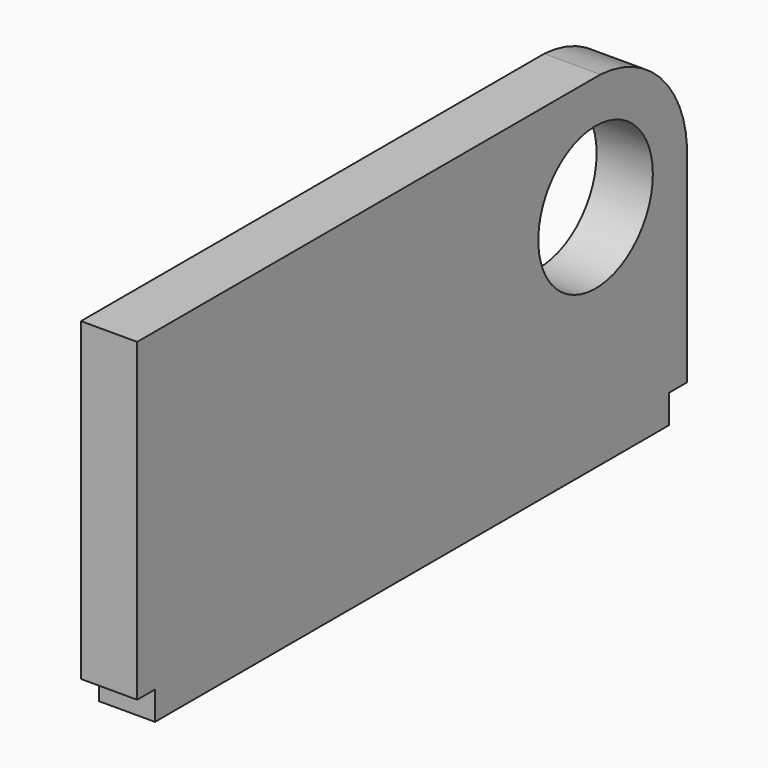
from build123d import *

# Parameters (mm, degrees)
F0_W     = 285.75
F0_H     = 12.7
F0_R     = 31.829375
F1_DEPTH = 25


# Not quite as in the source:
# - ends of sketch curves that miss each other by under 0.0002 mm in the source are joined


with BuildPart() as f1:
    # F0 (on Right) → F1 (new body)
    with BuildSketch(Plane.YZ):
        with Locations((-174.078946, 333.521804)):
            Rectangle(F0_W, F0_H)
        with BuildLine():
            Line((-316.953946, 339.871804), (-31.203946, 339.871804))
            Line((-31.203946, 339.871804), (-21.297946, 339.871804))
            Line((-21.297946, 339.871804), (-21.297946, 431.783595))
            ThreePointArc((-21.297946, 431.783595), (-36.138421464, 465.080578536), (-69.4354049904, 479.9210541806))
            Line((-69.4354049904, 479.9210541806), (-326.859946, 479.921054))
            Line((-326.859946, 479.921054), (-326.859946, 339.871804))
            Line((-326.859946, 339.871804), (-316.953946, 339.871804))
        make_face()
        with Locations((-72.140054, 429.078946)):
            Circle(F0_R, mode=Mode.SUBTRACT)
    extrude(amount=F1_DEPTH)


solid = f1.part
